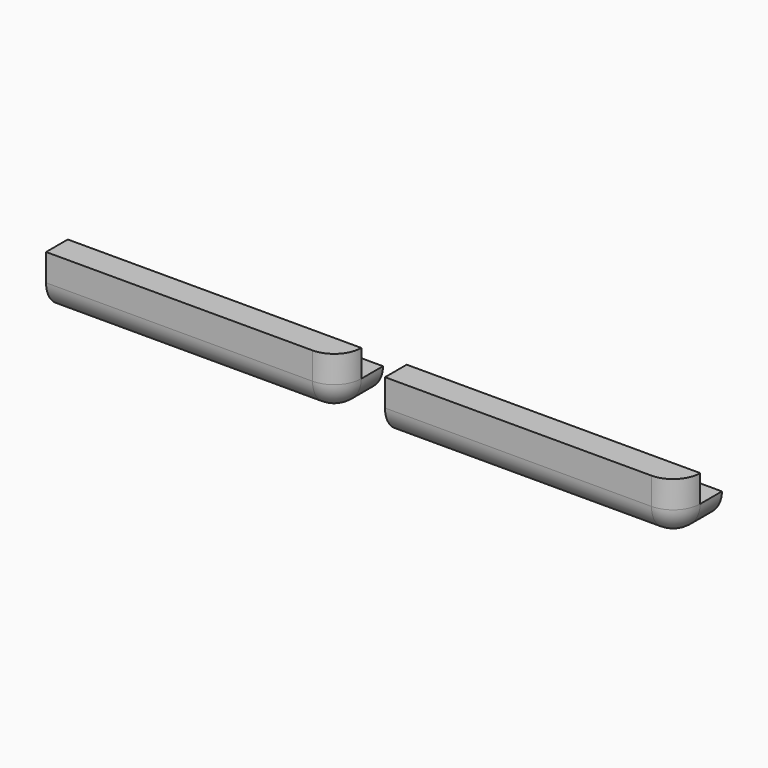
from build123d import *

# Parameters (mm, degrees)
F0_W     = 21.652942713
F0_H     = 2
F1_DEPTH = 4
F2_W     = 21.652942713
F2_H     = 2
F4_DEPTH = 2
F3_W     = 21.652942713
F3_H     = 2
F7_R     = 1.99999
F7_2_R   = 1.99999


# Not quite as in the source:
# - a fillet or chamfer is up to 0.001 mm smaller than in the source, because OpenCascade refuses the exact size


with BuildPart() as f1:
    # F0 (on Front) → F1 (new body)
    with BuildSketch(Plane.XZ):
        with Locations((-85.8919425884, 1)):
            Rectangle(F0_W, F0_H)
    extrude(amount=F1_DEPTH)


with BuildPart() as f1b:
    # F0 (on Front) → F1, piece 2 (new body)
    with BuildSketch(Plane.XZ):
        with Locations((85.8919425884, 1)):
            Rectangle(F0_W, F0_H)
    extrude(amount=F1_DEPTH)


with BuildPart() as f4:
    # F2 (on face) → F4 (new body)
    with BuildSketch(Plane.XY.offset(2)):
        with Locations((-85.8919425884, -3)):
            Rectangle(F2_W, F2_H)
    extrude(amount=F4_DEPTH)


with BuildPart() as f4b:
    # F3 (on face) → F4, piece 2 (new body)
    with BuildSketch(Plane.XY.offset(2)):
        with Locations((85.8919425884, -3)):
            Rectangle(F3_W, F3_H)
    extrude(amount=F4_DEPTH)


with BuildPart() as f1_1:
    add(f1.part)

    # F5: union F4
    add(f4.part)

    # F7 (radius 2 in the source; OpenCascade refuses exactly that, so slightly less here)
    f7_edges = [f1_1.edges().sort_by_distance(p)[0] for p in [
        (-96.718414, -2, 0),
        (-96.718414, -4, 2),
        (-85.891943, -4, 0),
        (-75.065471, -4, 2),
        (-75.065471, -2, 0),
    ]]
    fillet(f7_edges, radius=F7_R)


with BuildPart() as f1b_1:
    add(f1b.part)

    # F6: union F4b
    add(f4b.part)

    # F7#2 (radius 2 in the source; OpenCascade refuses exactly that, so slightly less here)
    f7_2_edges = [f1b_1.edges().sort_by_distance(p)[0] for p in [
        (96.718414, -2, 0),
        (96.718414, -4, 2),
        (85.891943, -4, 0),
    ]]
    fillet(f7_2_edges, radius=F7_2_R)


with BuildPart() as f9_1:
    # F9: copy of F1b
    add(f1b_1.part.moved(Location((-25, 0, 0))))


solid = Compound([f1b_1.part, f9_1.part])
